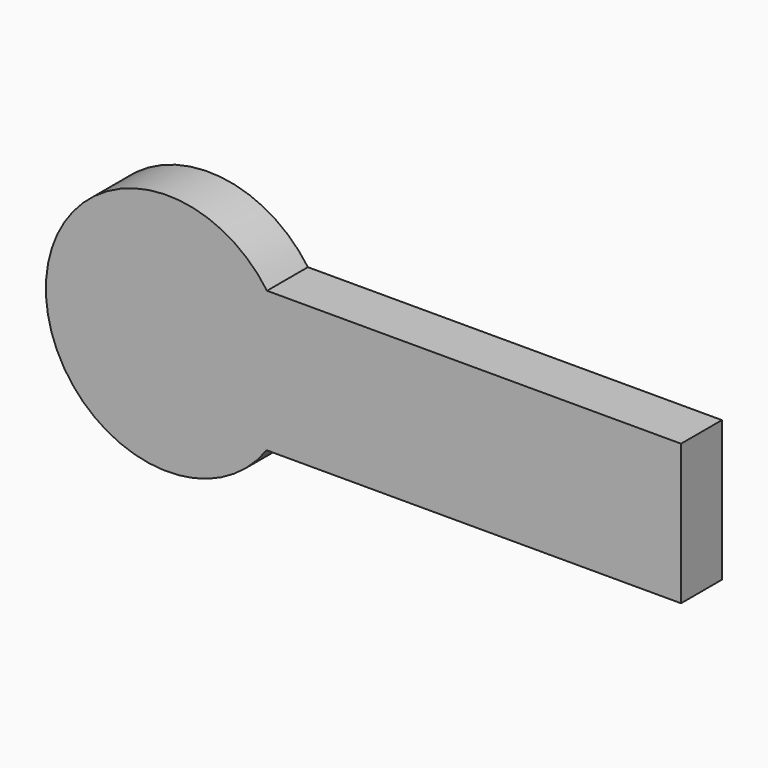
from build123d import *

# Parameters (mm, degrees)
F1_DEPTH = 25.4
F2_DEPTH = 25.4
F3_DEPTH = 25.4


with BuildPart() as f1:
    # F0 (on Front) → F1 (new body)
    with BuildSketch(Plane.XZ):
        with BuildLine():
            ThreePointArc((-119.86399662, 0), (-111.5302178098, 16.6558061897), (-108.6615478184, 35.0579387173))
            ThreePointArc((-108.6615478184, 35.0579387173), (-111.4781642304, 53.2963683876), (-119.6655722325, 69.8354129505))
            Line((-119.6655722325, 69.8354129505), (-201.6532506958, 69.8354129505))
            Line((-201.6532506958, 69.8354129505), (-201.6532506958, 0))
            Line((-201.6532506958, 0), (-119.86399662, 0))
        make_face()
        with BuildLine():
            ThreePointArc((-119.6655722325, 69.8354129505), (-111.4781642304, 53.2963683876), (-108.6615478184, 35.0579387173))
            ThreePointArc((-108.6615478184, 35.0579387173), (-111.5302178098, 16.6558061897), (-119.86399662, 0))
            Line((-119.86399662, 0), (86.1022950306, 0))
            Line((86.1022950306, 0), (86.1022950306, 69.8354129505))
            Line((86.1022950306, 69.8354129505), (-119.6655722325, 69.8354129505))
        make_face()
        with BuildLine():
            Line((-201.6532506958, 69.8354129505), (-119.6655722325, 69.8354129505))
            ThreePointArc((-119.6655722325, 69.8354129505), (-229.5771812139, 35.2297180557), (-119.86399662, 0))
            Line((-119.86399662, 0), (-201.6532506958, 0))
            Line((-201.6532506958, 0), (-201.6532506958, 69.8354129505))
        make_face()
    extrude(amount=F1_DEPTH)

    # F2 (add): a face of the model
    f2_faces = [f1.faces().sort_by_distance(p)[0] for p in [
        (-83.8129637721, 0, 34.9783538695),
    ]]
    extrude(f2_faces, amount=F2_DEPTH)

    # F3 (cut): a face of the model
    f3_faces = [f1.faces().sort_by_distance(p)[0] for p in [
        (-83.8129637721, -25.4, 34.9783538695),
    ]]
    extrude(f3_faces, amount=-F3_DEPTH, mode=Mode.SUBTRACT)


solid = f1.part
